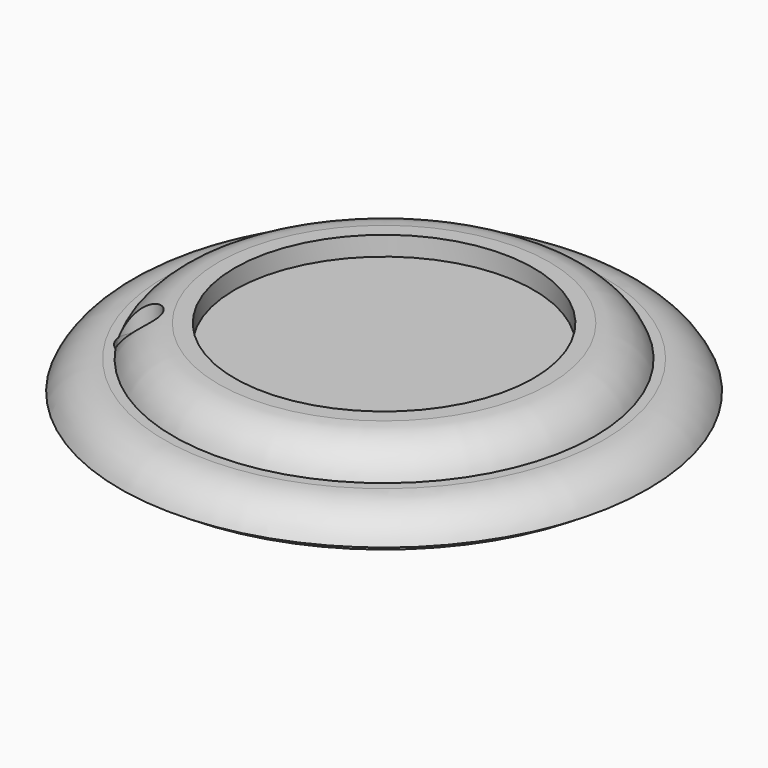
from build123d import *

# Parameters (mm, degrees)
F0_R      = 27.8603665739
F1_DEPTH  = 3.048
F4_R      = 26.2786257822
F5_DEPTH  = 1.016
F6_R      = 22.2176168744
F7_DEPTH  = 3.302
F9_R      = 15.773437446
F10_DEPTH = 2.032
F11_R     = 2.2956006308
F12_DEPTH = 21.336
F13_R     = 2.0464830212
F14_DEPTH = 25.4


# Not quite as in the source:
# - a fillet or chamfer that OpenCascade refuses, or shapes differently, is made with other operations: its cross-section is extruded or revolved along the edge and cut away or added


with BuildPart() as f1:
    # F0 (on Top) → F1 (new body)
    with BuildSketch(Plane.XY):
        Circle(F0_R)
    extrude(amount=F1_DEPTH)

    # F2: fillet of radius 5.08 on 1 edges, made by hand

    # F2_s1 → F2_t2 (revolve, cut)
    with BuildSketch(Plane.XZ):
        with BuildLine():
            ThreePointArc((27.8603665739, 0), (25.9869002599, 2.2182329348), (23.2044696678, 3.048))
            Line((23.2044696678, 3.048), (27.8603665739, 3.048))
            Line((27.8603665739, 3.048), (27.8603665739, 0))
        make_face()
    revolve(axis=Axis((0, 0, 3.048), (0, 0, 1)), mode=Mode.SUBTRACT)

    # F4 (on face) → F5 (join)
    with BuildSketch(Plane(origin=(0, 0, 0), x_dir=(1, 0, 0), z_dir=(0, 0, -1))):
        Circle(F4_R)
    extrude(amount=F5_DEPTH)

    # F6 (on face) → F7 (join)
    with BuildSketch(Plane.XY.offset(3.048)):
        Circle(F6_R)
    extrude(amount=F7_DEPTH)

    # F8: fillet of radius 5.08 on 1 edges, made by hand

    # F8_s1 → F8_t2 (revolve, cut)
    with BuildSketch(Plane.XZ):
        with BuildLine():
            ThreePointArc((22.2176168744, 3.048), (20.3549739793, 5.4436458882), (17.4589283996, 6.35))
            Line((17.4589283996, 6.35), (22.2176168744, 6.35))
            Line((22.2176168744, 6.35), (22.2176168744, 3.048))
        make_face()
    revolve(axis=Axis((0, 0, 6.35), (0, 0, 1)), mode=Mode.SUBTRACT)

    # F9 (on face) → F10 (cut)
    with BuildSketch(Plane.XY.offset(6.35)):
        Circle(F9_R)
    extrude(amount=-F10_DEPTH, mode=Mode.SUBTRACT)

    # F11 (on face) → F12 (cut)
    with BuildSketch(Plane.XY.offset(3.048)):
        with Locations((-17.1565320343, -10.5084851384)):
            Circle(F11_R)
    extrude(amount=-F12_DEPTH, mode=Mode.SUBTRACT)

    # F13 (on face) → F14 (cut)
    with BuildSketch(Plane.XY.offset(6.35)):
        with Locations((-17.3885338008, -10.6187639758)):
            Circle(F13_R)
    extrude(amount=-F14_DEPTH, mode=Mode.SUBTRACT)


solid = f1.part
